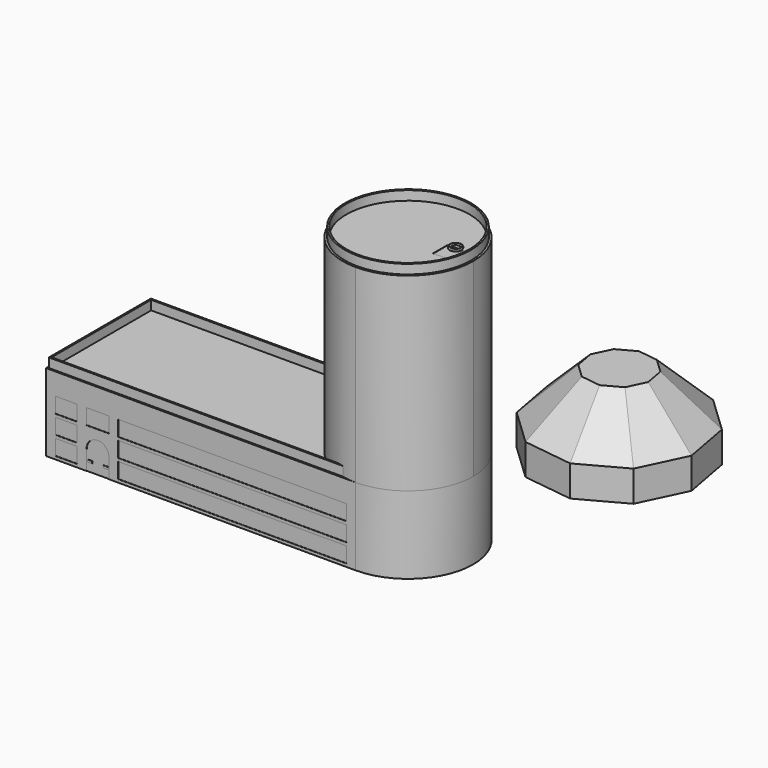
from build123d import *

# Parameters (mm, degrees)
F0_W        = 15
F0_H        = 15
F1_DEPTH    = 15
F2_W        = 2
F2_H        = 1
F2_W_2      = 1
F2_R        = 0.1684831901
F3_DEPTH    = 0.1
F4_W        = 17
F4_H        = 17
F4_W_2      = 15
F4_H_2      = 15
F5_DEPTH    = 10
F6_T1_DEPTH = 68.4336597593
F8_DEPTH    = 25
F10_DEPTH   = 61.2
F11_W       = 7.2363563826
F11_H       = 6.2551509271
F11_W_2     = 1.5
F11_H_2     = 0.75
F12_DEPTH   = 0.1
F13_R       = 20.4109975869
F13_R_2     = 19.8700915576
F14_DEPTH   = 3
F16_DEPTH   = 0.1
F18_DEPTH   = 0.5
F19_R       = 0.28
F20_W       = 7.0527685629
F20_H       = 5
F20_W_2     = 7.2363563826
F20_W_3     = 73.7108750545
F21_DEPTH   = 0.1
F23_DEPTH   = 3
F25_DEPTH   = 25
F26_SIZE    = 15


# Not quite as in the source:
# - a fillet or chamfer that OpenCascade refuses, or shapes differently, is made with other operations: its cross-section is extruded or revolved along the edge and cut away or added


with BuildPart() as f1:
    # F0 (on Top) → F1 (new body)
    with BuildSketch(Plane.XY):
        with Locations((-43.6317585409, 38.2814475718)):
            Rectangle(F0_W, F0_H)
    extrude(amount=F1_DEPTH)

    # F2 (on face) → F3 (cut)
    with BuildSketch(Plane.XZ.offset(-30.7814475718)):
        with Locations((-45.825777228, 3.4614248428)):
            Rectangle(F2_W, F2_H)
        with Locations((-48.325777228, 1.9614248428)):
            Rectangle(F2_W, F2_H)
        with Locations((-45.825777228, 1.9614248428)):
            Rectangle(F2_W, F2_H)
        with Locations((-47.7474738359, 6.606749177)):
            Rectangle(F2_W_2, F2_H)
        with Locations((-46.2474738359, 6.606749177)):
            Rectangle(F2_W_2, F2_H)
        with Locations((-47.7400628534, 8.106749177)):
            Rectangle(F2_W_2, F2_H)
        with Locations((-46.2474738359, 8.106749177)):
            Rectangle(F2_W_2, F2_H)
        with Locations((-40.9830439389, 8.106749177)):
            Rectangle(F2_W_2, F2_H)
        with Locations((-42.4830439389, 6.606749177)):
            Rectangle(F2_W_2, F2_H)
        with Locations((-40.9830439389, 6.606749177)):
            Rectangle(F2_W_2, F2_H)
        with BuildLine():
            ThreePointArc((-37.7868020667, 2.8161734808), (-38.9192876286, 3.9486590427), (-40.0517731905, 2.8161734808))
            Line((-40.0517731905, 2.8161734808), (-40.0517731905, 0))
            Line((-40.0517731905, 0), (-37.7868020667, 0))
            Line((-37.7868020667, 0), (-37.7868020667, 2.8161734808))
        make_face()
        with Locations((-38.3073501289, 1.4651020756)):
            Circle(F2_R, mode=Mode.SUBTRACT)
        with Locations((-48.325777228, 3.4614248428)):
            Rectangle(F2_W, F2_H)
        with Locations((-42.4830439389, 8.106749177)):
            Rectangle(F2_W_2, F2_H)
    extrude(amount=-F3_DEPTH, mode=Mode.SUBTRACT)

    # F4 (on face) → F5 (join)
    with BuildSketch(Plane.XY.offset(15)):
        with Locations((-43.6317585409, 38.2814475718)):
            Rectangle(F4_W, F4_H)
        with Locations((-43.6317585409, 38.2814475718)):
            Rectangle(F4_W_2, F4_H_2, mode=Mode.SUBTRACT)
        with Locations((-43.6317585409, 38.2814475718)):
            Rectangle(F4_W_2, F4_H_2)
    extrude(amount=F5_DEPTH)

    # F6: chamfer of 10 on 2 edges, made by hand

    # F6_s2 → F6_t1 (cut)
    with BuildSketch(Plane.XZ.offset(-72.4982774515)):
        Polygon((-52.1317585409, 15), (-42.1317585409, 25), (-52.1317585409, 25), align=None)
        Polygon((-35.1317585409, 15), (-45.1317585409, 25), (-35.1317585409, 25), align=None)
    extrude(amount=F6_T1_DEPTH, mode=Mode.SUBTRACT)


with BuildPart() as f8:
    # F7 (on Top) → F8 (new body)
    with BuildSketch(Plane.XY):
        with BuildLine():
            Line((27.3658934735, -18.1961677477), (-72.6341065265, -18.1961677477))
            Line((-72.6341065265, -18.1961677477), (-72.6341065265, -60.360345666))
            Line((-72.6341065265, -60.360345666), (27.3658934735, -60.360345666))
            ThreePointArc((27.3658934735, -60.360345666), (48.4479824327, -39.2782567069), (27.3658934735, -18.1961677477))
        make_face()
    extrude(amount=F8_DEPTH)

    # F9 (on face) → F10 (join)
    with BuildSketch(Plane.XY.offset(25)):
        with BuildLine():
            ThreePointArc((27.3658934735, -60.360345666), (42.2731815381, -54.1855447715), (48.4479824327, -39.2782567069))
            ThreePointArc((48.4479824327, -39.2782567069), (42.2731815381, -24.3709686423), (27.3658934735, -18.1961677477))
            ThreePointArc((27.3658934735, -18.1961677477), (6.2838045144, -39.2782567069), (27.3658934735, -60.360345666))
        make_face()
    extrude(amount=F10_DEPTH)

    # F11 (on face) → F12 (cut)
    with BuildSketch(Plane.XZ.offset(60.360345666)):
        with Locations((-55.9631597723, 3.1275754635)):
            Rectangle(F11_W, F11_H)
        with Locations((-58.5313379636, 3.0024008358)):
            Rectangle(F11_W_2, F11_H_2, mode=Mode.SUBTRACT)
        with Locations((-53.394981581, 3.0024008358)):
            Rectangle(F11_W_2, F11_H_2, mode=Mode.SUBTRACT)
        with BuildLine():
            ThreePointArc((-52.344981581, 6.2551509271), (-55.9631597723, 9.8733291184), (-59.5813379636, 6.2551509271))
            Line((-59.5813379636, 6.2551509271), (-52.344981581, 6.2551509271))
        make_face()
    extrude(amount=-F12_DEPTH, mode=Mode.SUBTRACT)

    # F13 (on face) → F14 (join)
    with BuildSketch(Plane.XY.offset(86.2)):
        with Locations((27.3658934735, -39.2782567069)):
            Circle(F13_R)
        with Locations((27.3658934735, -39.2782567069)):
            Circle(F13_R_2, mode=Mode.SUBTRACT)
    extrude(amount=F14_DEPTH)

    # F15 (on face) → F16 (cut)
    with BuildSketch(Plane.XY.offset(86.2)):
        with BuildLine():
            ThreePointArc((38.9867735619, -36.2862572074), (40.3608889878, -37.6603726333), (41.7350044137, -36.2862572074))
            Line((41.7350044137, -36.2862572074), (38.9867735619, -36.2862572074))
        make_face()
        with BuildLine():
            Line((42.8608889878, -36.2862572074), (42.2988002924, -36.2862572074))
            ThreePointArc((42.2988002924, -36.2862572074), (40.3608889878, -38.2241685121), (38.4229776831, -36.2862572074))
            Line((38.4229776831, -36.2862572074), (37.8608889878, -36.2862572074))
            Line((37.8608889878, -36.2862572074), (37.8608889878, -42.2862572074))
            Line((37.8608889878, -42.2862572074), (42.8608889878, -42.2862572074))
            Line((42.8608889878, -42.2862572074), (42.8608889878, -36.2862572074))
        make_face()
    extrude(amount=-F16_DEPTH, mode=Mode.SUBTRACT)

    # F17 (on face) → F18 (join)
    with BuildSketch(Plane.XY.offset(86.2)):
        with BuildLine():
            ThreePointArc((38.4229776831, -36.2862572074), (40.3608889878, -38.2241685121), (42.2988002924, -36.2862572074))
            ThreePointArc((42.2988002924, -36.2862572074), (40.3608889878, -34.3483459027), (38.4229776831, -36.2862572074))
        make_face()
        with BuildLine():
            ThreePointArc((38.9867735619, -36.2862572074), (40.3608889878, -34.9121417815), (41.7350044137, -36.2862572074))
            ThreePointArc((41.7350044137, -36.2862572074), (40.3608889878, -37.6603726333), (38.9867735619, -36.2862572074))
        make_face(mode=Mode.SUBTRACT)
    extrude(amount=F18_DEPTH)

    # F19
    f19_edges = [f8.edges().sort_by_distance(p)[0] for p in [
        (42.2988, -36.286257, 86.7),
        (41.735004, -36.286257, 86.7),
    ]]
    fillet(f19_edges, radius=F19_R)

    # F20 (on face) → F21 (cut)
    with BuildSketch(Plane.XZ.offset(60.360345666)):
        with Locations((-66.107722245, 3.5)):
            Rectangle(F20_W, F20_H)
        with Locations((-66.107722245, 9.5)):
            Rectangle(F20_W, F20_H)
        with Locations((-66.107722245, 15.5)):
            Rectangle(F20_W, F20_H)
        with Locations((-55.9631597723, 15.5)):
            Rectangle(F20_W_2, F20_H)
        with Locations((-12.4895440537, 15.5)):
            Rectangle(F20_W_3, F20_H)
        with Locations((-12.4895440537, 9.5)):
            Rectangle(F20_W_3, F20_H)
        with Locations((-12.4895440537, 3.5)):
            Rectangle(F20_W_3, F20_H)
    extrude(amount=-F21_DEPTH, mode=Mode.SUBTRACT)

    # F22 (on face) → F23 (join)
    with BuildSketch(Plane.XY.offset(25)):
        with BuildLine():
            Line((22.801675144, -18.6961677477), (-72.1341065265, -18.6961677477))
            Line((-72.1341065265, -18.6961677477), (-72.1341065265, -59.860345666))
            Line((-72.1341065265, -59.860345666), (22.801675144, -59.860345666))
            ThreePointArc((22.801675144, -59.860345666), (21.8701293813, -59.6314149858), (20.9499619029, -59.360345666))
            Line((20.9499619029, -59.360345666), (-71.6341065265, -59.360345666))
            Line((-71.6341065265, -59.360345666), (-71.6341065265, -19.1961677477))
            Line((-71.6341065265, -19.1961677477), (20.9499619029, -19.1961677477))
            ThreePointArc((20.9499619029, -19.1961677477), (21.8701293813, -18.925098428), (22.801675144, -18.6961677477))
        make_face()
    extrude(amount=F23_DEPTH)


with BuildPart() as f25:
    # F24 (on Top) → F25 (new body)
    with BuildSketch(Plane.XY):
        Polygon((51.5826063814, 53.6310353183), (35.4753058491, 55.7492638375), (21.1991625003, 47.9953130003), (14.2071778661, 33.3309284795), (17.1700524279, 17.3574067378), (28.9560688076, 6.1760901607), (45.06336934, 4.0578616415), (59.3395126887, 11.8118124787), (66.3314973229, 26.4761969995), (63.3686227611, 42.4497187412), align=None)
    extrude(amount=F25_DEPTH)

    # F26
    f26_edges = [f25.edges().sort_by_distance(p)[0] for p in [
        (62.835505, 19.144005, 25),
        (64.85006, 34.462958, 25),
        (57.475615, 48.040377, 25),
        (43.528956, 54.69015, 25),
        (28.337234, 51.872288, 25),
        (17.70317, 40.663121, 25),
        (23.063061, 11.766748, 25),
        (37.009719, 5.116976, 25),
        (52.201441, 7.934837, 25),
        (15.688615, 25.344168, 25),
    ]]
    chamfer(f26_edges, length=F26_SIZE)


solid = Compound([f1.part, f8.part, f25.part])
